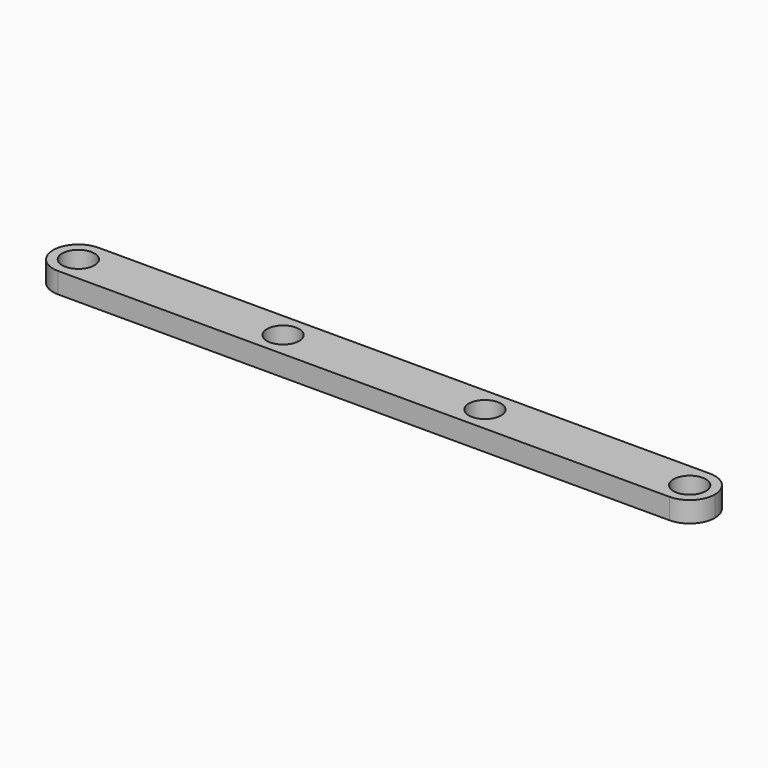
from build123d import *

# Parameters (mm, degrees)
F0_W     = 104.1019
F0_H     = 7.9375
F0_R     = 2.54
F1_DEPTH = 3.2512
F2_R     = 3.96874


# Not quite as in the source:
# - a fillet or chamfer is up to 0.001 mm smaller than in the source, because OpenCascade refuses the exact size


with BuildPart() as f1:
    # F0 (on Top) → F1 (new body)
    with BuildSketch(Plane.XY):
        with Locations((52.05095, -3.96875)):
            Rectangle(F0_W, F0_H)
        with Locations((3.96875, -3.96875)):
            Circle(F0_R, mode=Mode.SUBTRACT)
        with Locations((36.17595, -3.96875)):
            Circle(F0_R, mode=Mode.SUBTRACT)
        with Locations((67.92595, -3.96875)):
            Circle(F0_R, mode=Mode.SUBTRACT)
        with Locations((100.13315, -3.96875)):
            Circle(F0_R, mode=Mode.SUBTRACT)
    extrude(amount=F1_DEPTH)

    # F2 (radius 3.96875 in the source; OpenCascade refuses exactly that, so slightly less here)
    f2_edges = [f1.edges().sort_by_distance(p)[0] for p in [
        (0, 0, 1.6256),
        (0, -7.9375, 1.6256),
        (104.1019, -7.9375, 1.6256),
        (104.1019, 0, 1.6256),
    ]]
    fillet(f2_edges, radius=F2_R)


solid = f1.part
